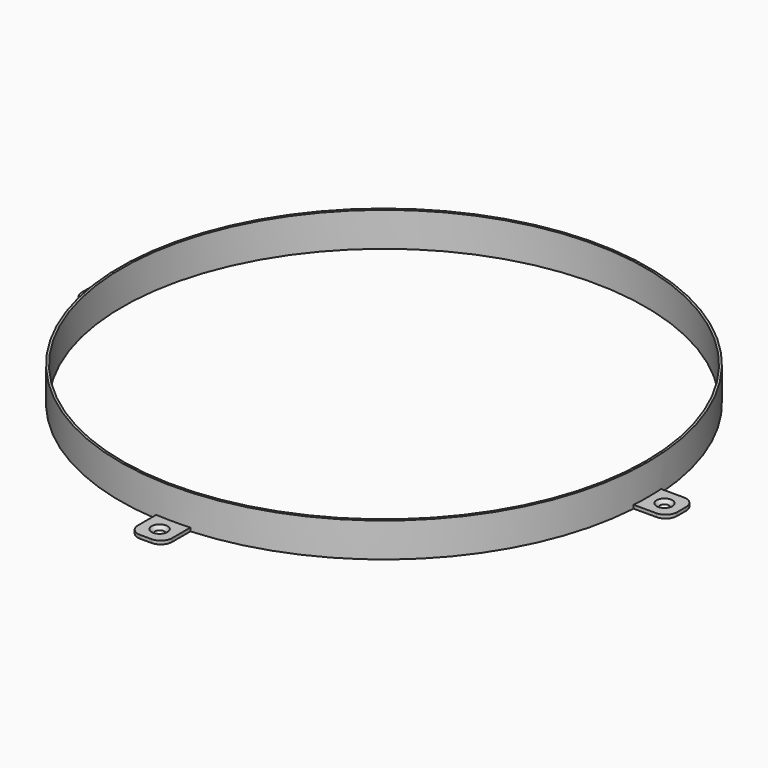
from build123d import *

# Parameters (mm, degrees)
F0_R     = 231
F0_R_2   = 229
F1_DEPTH = 30
F2_W     = 30
F2_H     = 30
F3_DEPTH = 3
F4_R     = 4
F5_DEPTH = 25
F6_R     = 10
F8_COUNT = 4
F9_SIZE  = 2.99999


# Not quite as in the source:
# - a fillet or chamfer is up to 0.001 mm smaller than in the source, because OpenCascade refuses the exact size


with BuildPart() as f1:
    # F0 (on Top) → F1 (new body)
    with BuildSketch(Plane.XY):
        Circle(F0_R)
        Circle(F0_R_2, mode=Mode.SUBTRACT)
    extrude(amount=F1_DEPTH)

    # F2 (on face) → F3 (join)
    with BuildSketch(Plane(origin=(0, 0, 0), x_dir=(1, 0, 0), z_dir=(0, 0, -1))):
        with Locations((0, -245.5124725476)):
            Rectangle(F2_W, F2_H)
    extrude(amount=-F3_DEPTH)

    # F4 (on face) → F5 (cut)
    with BuildSketch(Plane(origin=(0, 0, 0), x_dir=(1, 0, 0), z_dir=(0, 0, -1))):
        with Locations((0, -245.5124725476)):
            Circle(F4_R)
    extrude(amount=-F5_DEPTH, mode=Mode.SUBTRACT)

    # F6
    f6_edges = [f1.edges().sort_by_distance(p)[0] for p in [
        (-15, 260.512473, 1.5),
        (15, 260.512473, 1.5),
    ]]
    fillet(f6_edges, radius=F6_R)

    # F8: F1 ×4 about axis
    f8_axis = Axis((0, 0, -51.1162020266), (0, 0, -1))


with BuildPart() as f1_1:
    add(f1.part)
    for i in range(1, F8_COUNT):
        add(f1.part.rotate(f8_axis, i * 360 / F8_COUNT))

    # F9 (size 3 in the source; OpenCascade refuses exactly that, so slightly less here)
    f9_edges = [f1_1.edges().sort_by_distance(p)[0] for p in [
        (-245.512473, -4, 3),
        (-4, 245.512473, 3),
        (245.512473, 4, 3),
        (4, -245.512473, 3),
    ]]
    chamfer(f9_edges, length=F9_SIZE)


solid = f1_1.part
